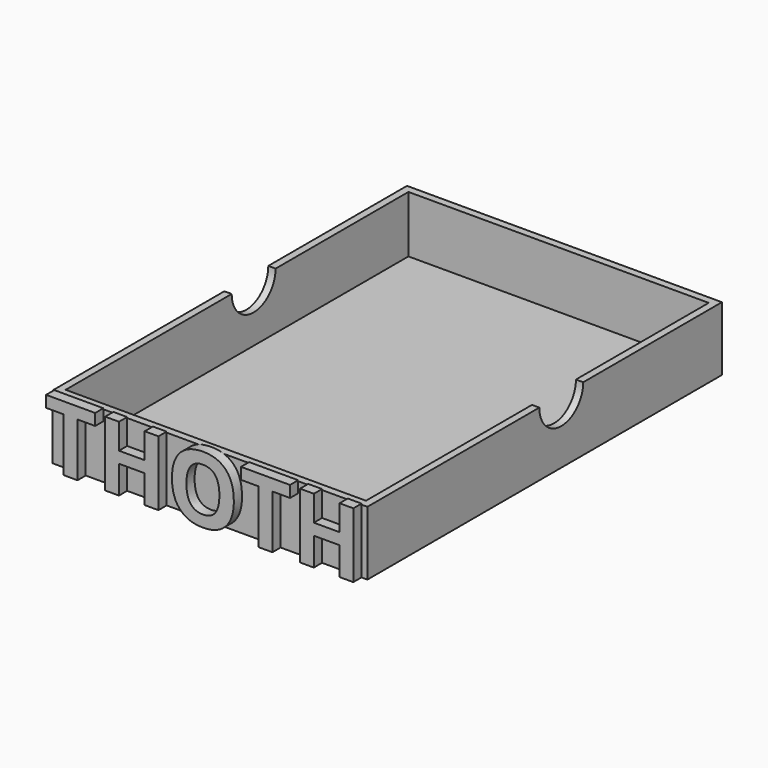
from build123d import *

# Parameters (mm, degrees)
F0_W         = 109.22
F0_H         = 153.67
F1_DEPTH     = 22.225
F2_T         = -2.54
F4_D         = 19.05
F5_TEXT_SIZE = 31.5764557076
F6_DEPTH     = 3.556


# Not quite as in the source:
# - Text() gives the source's letters only with a copy of the font that has no kerning and outlines rounded to 1/6400 em; it was checked with that copy


with BuildPart() as f1:
    # F0 (on Top) → F1 (new body)
    with BuildSketch(Plane.XY):
        with Locations((-9.645473212, -7.1984927896)):
            Rectangle(F0_W, F0_H)
    extrude(amount=F1_DEPTH)

    # F2
    f2_openings = [f1.faces().sort_by_distance(p)[0] for p in [
        (-9.645473, -7.198493, 22.225),
    ]]
    offset(amount=F2_T, openings=f2_openings)

    # F4 (through all)
    with Locations(Plane.YZ.offset(44.964526788)):
        with Locations((0, 22.225)):
            Hole(F4_D / 2)

    # F5 (on face) → F6 (join)
    with BuildSketch(Plane.XZ.offset(84.0334927896)):
        with Locations((-64.255473212, 0)):
            Text('THOTH', F5_TEXT_SIZE, font='Open Sans', font_style=FontStyle.BOLD, text_align=(TextAlign.LEFT, TextAlign.BOTTOM))
    extrude(amount=F6_DEPTH)


solid = f1.part
